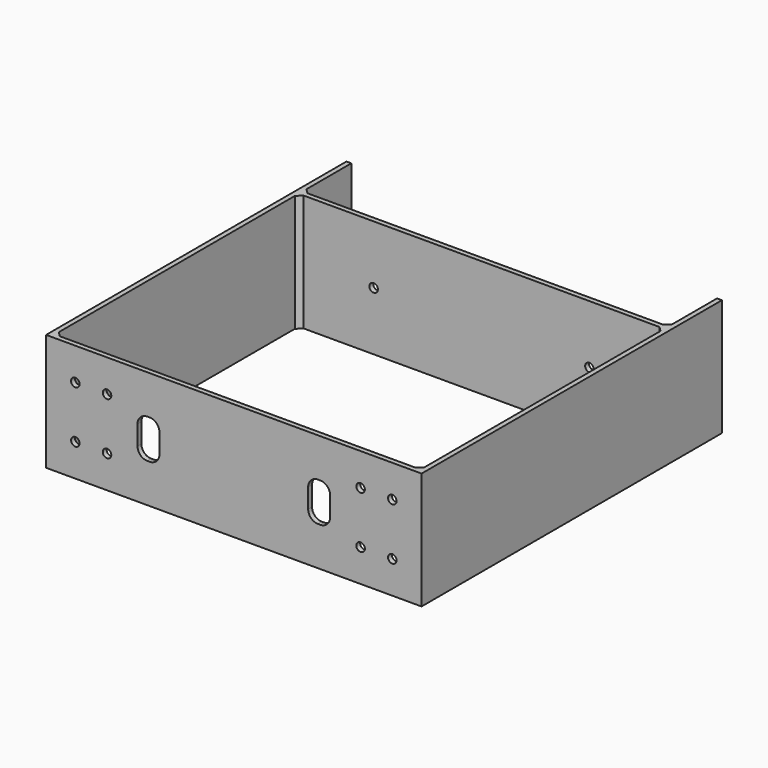
from build123d import *

# Parameters (mm, degrees)
F0_W     = 150
F0_H     = 125
F1_DEPTH = 48
F2_R     = 1.75
F2_W     = 9
F2_H     = 16
F3_DEPTH = 2
F4_R     = 1.75
F5_DEPTH = 2
F6_SIZE  = 2
F7_R     = 4


with BuildPart() as f1:
    # F0 (on Top) → F1 (new body)
    with BuildSketch(Plane.XY):
        Polygon((75, 89.5), (75, 64.5), (-75, 64.5), (-75, 89.5), (-77, 89.5), (-77, 64.5), (-77, -64.5), (77, -64.5), (77, 64.5), (77, 89.5), align=None)
        Rectangle(F0_W, F0_H, mode=Mode.SUBTRACT)
    extrude(amount=F1_DEPTH)

    # F2 (on face) → F3 (cut)
    with BuildSketch(Plane.XZ.offset(64.5)):
        with Locations((-65, 34.7)):
            Circle(F2_R)
        with Locations((-52, 34.7)):
            Circle(F2_R)
        with Locations((-65, 13.3)):
            Circle(F2_R)
        with Locations((-52, 13.3)):
            Circle(F2_R)
        with Locations((52, 34.7)):
            Circle(F2_R)
        with Locations((65, 34.7)):
            Circle(F2_R)
        with Locations((52, 13.3)):
            Circle(F2_R)
        with Locations((65, 13.3)):
            Circle(F2_R)
        with Locations((-35, 24)):
            Rectangle(F2_W, F2_H)
        with Locations((35, 24)):
            Rectangle(F2_W, F2_H)
    extrude(amount=-F3_DEPTH, mode=Mode.SUBTRACT)

    # F4 (on face) → F5 (cut)
    with BuildSketch(Plane.XZ.offset(-62.5)):
        with Locations((-44.25, 24)):
            Circle(F4_R)
        with Locations((44.25, 24)):
            Circle(F4_R)
    extrude(amount=-F5_DEPTH, mode=Mode.SUBTRACT)

    # F6
    f6_edges = [f1.edges().sort_by_distance(p)[0] for p in [
        (-75, 62.5, 24),
        (-75, -62.5, 24),
        (75, -62.5, 24),
        (75, 62.5, 24),
        (75, 64.5, 24),
        (-75, 64.5, 24),
    ]]
    chamfer(f6_edges, length=F6_SIZE)

    # F7
    f7_edges = [f1.edges().sort_by_distance(p)[0] for p in [
        (-39.5, -63.5, 16),
        (-30.5, -63.5, 16),
        (-30.5, -63.5, 32),
        (-39.5, -63.5, 32),
        (30.5, -63.5, 16),
        (39.5, -63.5, 16),
        (39.5, -63.5, 32),
        (30.5, -63.5, 32),
    ]]
    fillet(f7_edges, radius=F7_R)


solid = f1.part
